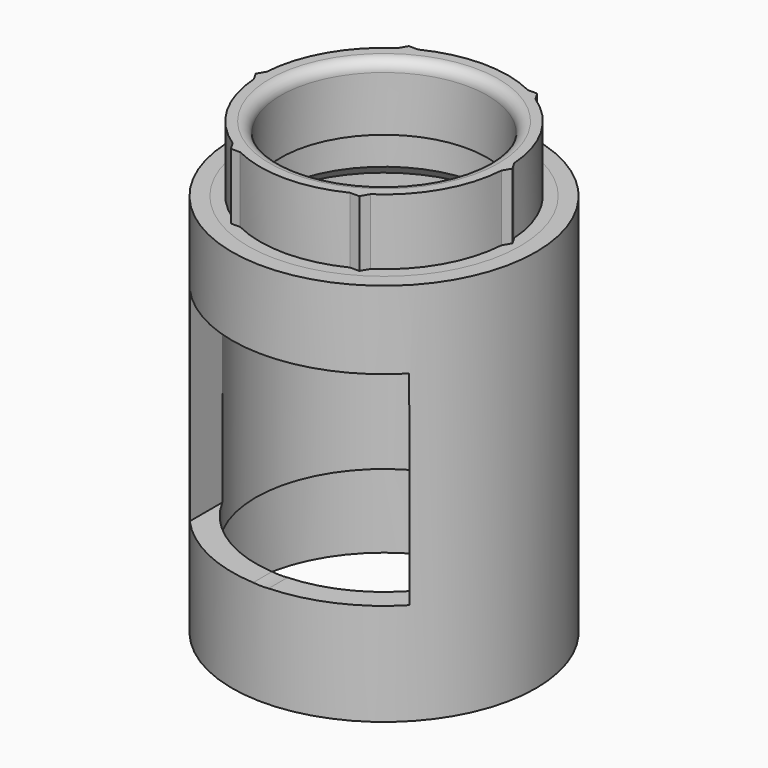
from build123d import *

# Parameters (mm, degrees)
F0_R      = 13.85
F0_R_2    = 11.7
F1_DEPTH  = 35
F2_R      = 9.4254173389
F3_DEPTH  = 6
F4_R      = 12.3979909048
F4_R_2    = 10.2650176462
F5_DEPTH  = 4
F6_SIZE   = 1
F7_R      = 1
F8_R      = 12.25
F9_DEPTH  = 7
F12_DEPTH = 13
F14_DEPTH = 10


with BuildPart() as f1:
    # F0 (on Top) → F1 (new body)
    with BuildSketch(Plane.XY):
        Circle(F0_R)
        Circle(F0_R_2, mode=Mode.SUBTRACT)
    extrude(amount=F1_DEPTH)

    # F8 (on face) → F9 (cut)
    with BuildSketch(Plane(origin=(0, 0, 0), x_dir=(1, 0, 0), z_dir=(0, 0, -1))):
        Circle(F8_R)
    extrude(amount=-F9_DEPTH, mode=Mode.SUBTRACT)

    # F11 (on offset) → F12 (cut)
    with BuildSketch(Plane.XZ.offset(14)):
        Polygon((9.9823940545, 25), (-10.2992961183, 25), (-10.2992961183, 17.1566890553), (-10.2992961183, 9.3133781105), (-0.8714802098, 9.3133781105), (0.554578146, 9.3133781105), (9.9823940545, 9.3133781105), (9.9823940545, 17.1566890553), align=None)
        with BuildLine():
            Line((0.554578146, 9.3133781105), (-0.8714802098, 9.3133781105))
            ThreePointArc((-0.8714802098, 9.3133781105), (-0.1584510319, 9.2890687527), (0.554578146, 9.3133781105))
        make_face()
    extrude(amount=-F12_DEPTH, mode=Mode.SUBTRACT)

    # F13 (on offset) → F14 (cut)
    with BuildSketch(Plane.XZ.offset(14)):
        Polygon((-10.2992961183, 27.9020555317), (-10.2992961183, 25), (9.9823940545, 25), (9.9626844749, 27.9020555317), align=None)
    extrude(amount=-F14_DEPTH, mode=Mode.SUBTRACT)


with BuildPart() as f3:
    # F2 (on face) → F3 (new body)
    with BuildSketch(Plane.XY.offset(35)):
        with BuildLine():
            ThreePointArc((11.276124747, -0.7341734743), (11.2940296095, -0.3672807911), (11.3, 0))
            ThreePointArc((11.3, 0), (11.2940296095, 0.3672807911), (11.276124747, 0.7341734743))
            Line((11.276124747, 0.7341734743), (6.273875253, 9.39832375))
            ThreePointArc((6.273875253, 9.39832375), (5.65, 9.7860870628), (5.002249494, 10.1324972243))
            Line((5.002249494, 10.1324972243), (-5.002249494, 10.1324972243))
            ThreePointArc((-5.002249494, 10.1324972243), (-5.65, 9.7860870628), (-6.273875253, 9.39832375))
            Line((-6.273875253, 9.39832375), (-11.276124747, 0.7341734743))
            ThreePointArc((-11.276124747, 0.7341734743), (-11.3, 0), (-11.276124747, -0.7341734743))
            Line((-11.276124747, -0.7341734743), (-6.273875253, -9.39832375))
            ThreePointArc((-6.273875253, -9.39832375), (-5.65, -9.7860870628), (-5.002249494, -10.1324972243))
            Line((-5.002249494, -10.1324972243), (5.002249494, -10.1324972243))
            ThreePointArc((5.002249494, -10.1324972243), (5.65, -9.7860870628), (6.273875253, -9.39832375))
            Line((6.273875253, -9.39832375), (11.276124747, -0.7341734743))
        make_face()
        Circle(F2_R, mode=Mode.SUBTRACT)
        with BuildLine():
            ThreePointArc((11.276124747, 0.7341734743), (11.2940296095, 0.3672807911), (11.3, 0))
            ThreePointArc((11.3, 0), (11.2940296095, -0.3672807911), (11.276124747, -0.7341734743))
            Line((11.276124747, -0.7341734743), (11.7, 0))
            Line((11.7, 0), (11.276124747, 0.7341734743))
        make_face()
        with BuildLine():
            Line((6.273875253, 9.39832375), (11.276124747, 0.7341734743))
            ThreePointArc((11.276124747, 0.7341734743), (9.7860870628, 5.65), (6.273875253, 9.39832375))
        make_face()
        with BuildLine():
            ThreePointArc((6.273875253, -9.39832375), (9.7860870628, -5.65), (11.276124747, -0.7341734743))
            Line((11.276124747, -0.7341734743), (6.273875253, -9.39832375))
        make_face()
        with BuildLine():
            ThreePointArc((5.002249494, 10.1324972243), (5.65, 9.7860870628), (6.273875253, 9.39832375))
            Line((6.273875253, 9.39832375), (5.85, 10.1324972243))
            Line((5.85, 10.1324972243), (5.002249494, 10.1324972243))
        make_face()
        with BuildLine():
            Line((5.85, -10.1324972243), (6.273875253, -9.39832375))
            ThreePointArc((6.273875253, -9.39832375), (5.65, -9.7860870628), (5.002249494, -10.1324972243))
            Line((5.002249494, -10.1324972243), (5.85, -10.1324972243))
        make_face()
        with BuildLine():
            Line((-5.002249494, 10.1324972243), (5.002249494, 10.1324972243))
            ThreePointArc((5.002249494, 10.1324972243), (0, 11.3), (-5.002249494, 10.1324972243))
        make_face()
        with BuildLine():
            ThreePointArc((-5.002249494, -10.1324972243), (0, -11.3), (5.002249494, -10.1324972243))
            Line((5.002249494, -10.1324972243), (-5.002249494, -10.1324972243))
        make_face()
        with BuildLine():
            ThreePointArc((-6.273875253, 9.39832375), (-5.65, 9.7860870628), (-5.002249494, 10.1324972243))
            Line((-5.002249494, 10.1324972243), (-5.85, 10.1324972243))
            Line((-5.85, 10.1324972243), (-6.273875253, 9.39832375))
        make_face()
        with BuildLine():
            Line((-5.85, -10.1324972243), (-5.002249494, -10.1324972243))
            ThreePointArc((-5.002249494, -10.1324972243), (-5.65, -9.7860870628), (-6.273875253, -9.39832375))
            Line((-6.273875253, -9.39832375), (-5.85, -10.1324972243))
        make_face()
        with BuildLine():
            Line((-11.276124747, 0.7341734743), (-6.273875253, 9.39832375))
            ThreePointArc((-6.273875253, 9.39832375), (-9.7860870628, 5.65), (-11.276124747, 0.7341734743))
        make_face()
        with BuildLine():
            ThreePointArc((-11.276124747, -0.7341734743), (-9.7860870628, -5.65), (-6.273875253, -9.39832375))
            Line((-6.273875253, -9.39832375), (-11.276124747, -0.7341734743))
        make_face()
        with BuildLine():
            ThreePointArc((-11.276124747, -0.7341734743), (-11.3, 0), (-11.276124747, 0.7341734743))
            Line((-11.276124747, 0.7341734743), (-11.7, 0))
            Line((-11.7, 0), (-11.276124747, -0.7341734743))
        make_face()
    extrude(amount=F3_DEPTH)

    # F4 (on face) → F5 (join)
    with BuildSketch(Plane.XY.offset(35)):
        Circle(F4_R)
        Circle(F4_R_2, mode=Mode.SUBTRACT)
    extrude(amount=-F5_DEPTH)

    # F6
    f6_edges = [f3.edges().sort_by_distance(p)[0] for p in [
        (-10.265018, 0, 31),
    ]]
    chamfer(f6_edges, length=F6_SIZE)

    # F7
    f7_edges = [f3.edges().sort_by_distance(p)[0] for p in [
        (-9.425417, 0, 41),
    ]]
    fillet(f7_edges, radius=F7_R)


solid = Compound([f1.part, f3.part])
